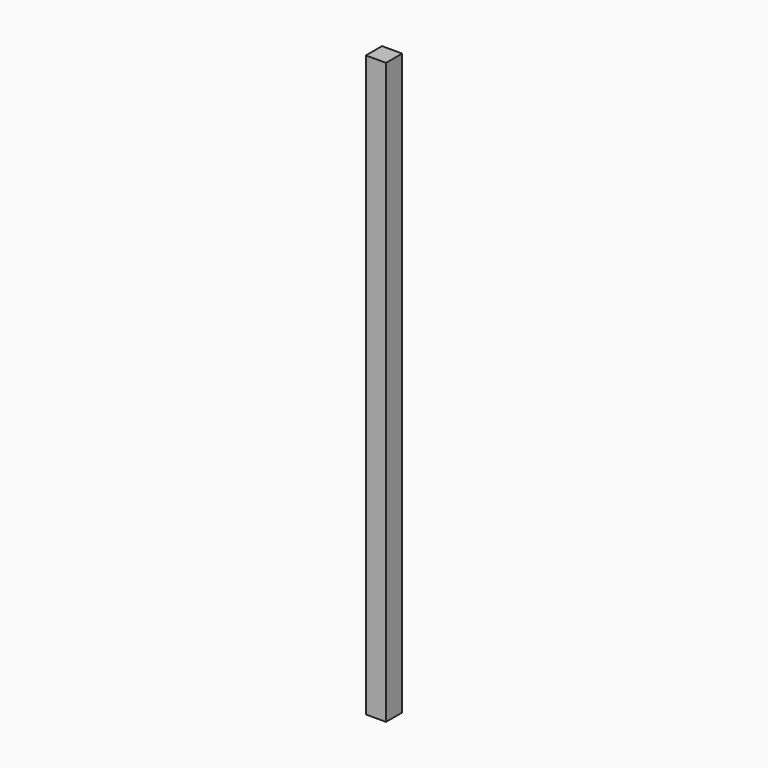
from build123d import *

# Parameters (mm, degrees)
F0_W     = 80
F0_H     = 80
F1_DEPTH = 2300


# Not quite as in the source:
# - a feature names something its author has since deleted; it is built from what else it names


with BuildPart() as f1:
    # F0 (on Top) → F1 (new body)
    with BuildSketch(Plane.XY):
        with Locations((-5.0000006985, -15.3164538797)):
            Rectangle(F0_W, F0_H)
    extrude(amount=F1_DEPTH)


solid = f1.part
